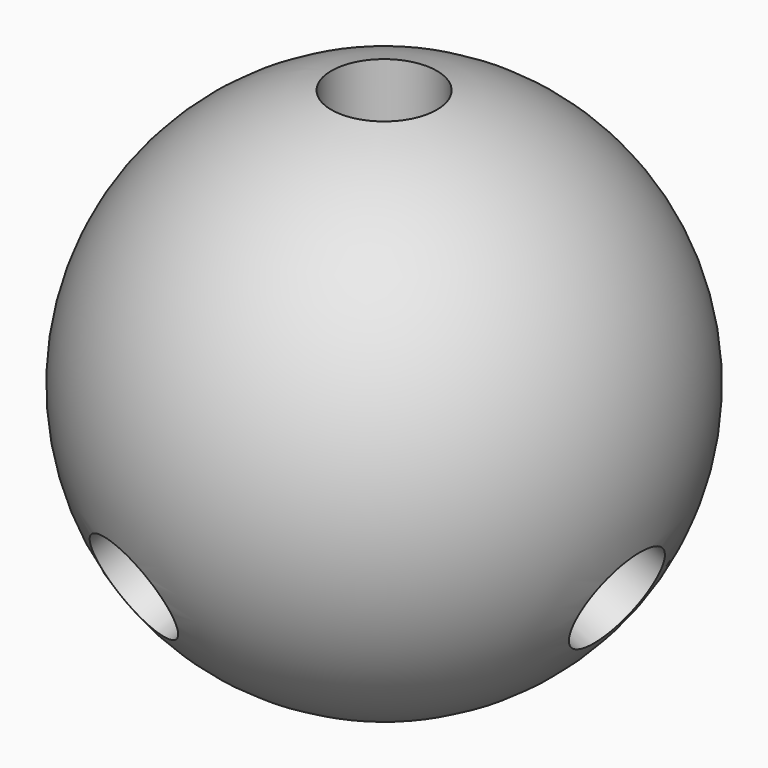
from build123d import *

# Parameters (mm, degrees)
F5_R      = 3.175
F6_DEPTH  = 50.8
F9_ANGLE  = 115.8
F10_ANGLE = 108.4
F11_ANGLE = 107.7


# Not quite as in the source:
# - a length typed as a fraction of an inch, garbled in the dataset ("3 / 203.2 mm" for 3/8 in), is restored


with BuildPart() as f2:
    # F0 (on Front) → F2 (revolve)
    with BuildSketch(Plane.XZ):
        with BuildLine():
            Line((0, -15.875), (0, 15.875))
            ThreePointArc((0, 15.875), (-15.875, 0), (0, -15.875))
        make_face()
    revolve(axis=Axis((0, 0, 0), (0, 0, 1)))


with BuildPart() as f6:
    # F5 (on offset) → F6 (new body)
    with BuildSketch(Plane.XY.offset(5.715)):
        Circle(F5_R)
    extrude(amount=F6_DEPTH)


with BuildPart() as f9_1:
    # F9: copy of F6
    add(f6.part.rotate(Axis((0, 33.8576585054, 0), (0, 1, 0)), F9_ANGLE))


with BuildPart() as f10_1:
    # F10: copy of F9_1
    add(f9_1.part.rotate(Axis((0, 0, -28.0886162072), (0, 0, -1)), F10_ANGLE))


with BuildPart() as f11_1:
    # F11: copy of F10_1
    add(f10_1.part.rotate(Axis((0, 0, -28.0886162072), (0, 0, -1)), F11_ANGLE))


with BuildPart() as f2_1:
    add(f2.part)

    # F12: cut F6, F10_1, F11_1, F9_1
    add(f6.part, mode=Mode.SUBTRACT)
    add(f10_1.part, mode=Mode.SUBTRACT)
    add(f11_1.part, mode=Mode.SUBTRACT)
    add(f9_1.part, mode=Mode.SUBTRACT)


solid = f2_1.part
